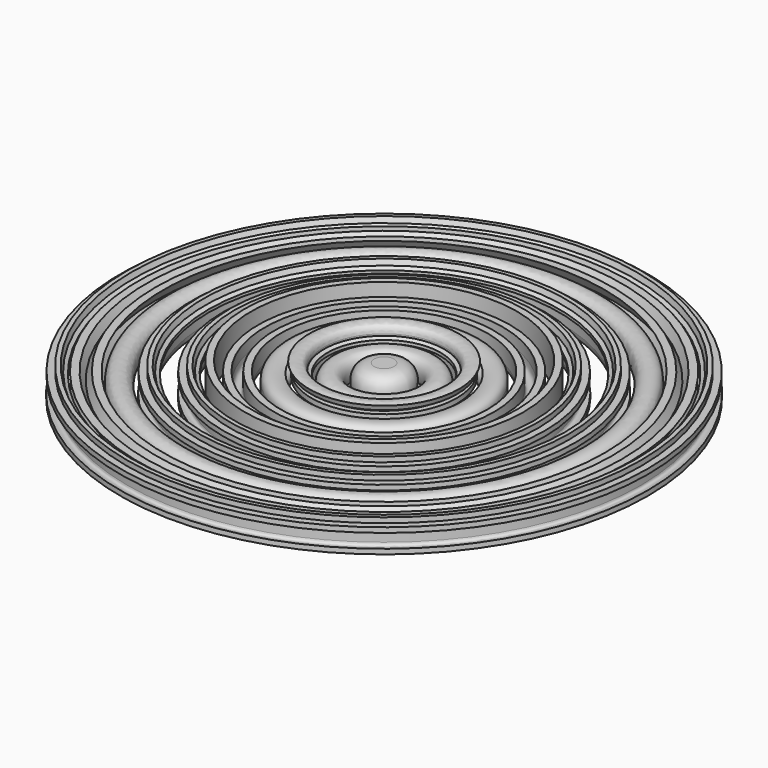
from build123d import *

# Parameters (mm, degrees)
F0_TEXT_SIZE = 64.0149060119
F1_DEPTH     = 25.4
F1_FACE_W    = 9.5322195983
F1_FACE_H    = 48.64132624


# Not quite as in the source:
# - Text() gives the source's letters only with a copy of the font that has no kerning and outlines rounded to 1/6400 em; it was checked with that copy


with BuildPart() as f1:
    # F0 (on Front) → F1 (new body)
    with BuildSketch(Plane.XZ):
        with Locations((-95.4079255462, 3.5789469257)):
            Text('Default text', F0_TEXT_SIZE, font='Open Sans', font_style=FontStyle.BOLD, text_align=(TextAlign.LEFT, TextAlign.BOTTOM))
    extrude(amount=F1_DEPTH)


with BuildPart() as f2:
    # F1_face (on face) → F2 (revolve)
    with BuildSketch(Plane(origin=(-72.8163367303, 0, 26.4794588541), x_dir=(1, 0, 0), z_dir=(0, 1, 0))):
        with BuildLine():
            add(Edge.make_bspline(
                [(-3.8972357946, 22.9005119284), (8.2255870314, 22.9005119284), (21.0785798791, 10.8977170511), (21.0785798791, -10.9873789417), (8.6956964974, -22.8001295667), (-2.4969097256, -22.8001295667)],
                knots=[0, 0, 0, 1, 2, 2.9397163121, 3.8794326241, 3.8794326241, 3.8794326241], degree=2))
            Line((-3.8972357946, 22.9005119284), (-16.8402496039, 22.9005119284))
            Line((-16.8402496039, 22.9005119284), (-16.8402496039, -22.8001295667))
            Line((-16.8402496039, -22.8001295667), (-2.4969097256, -22.8001295667))
        make_face()
        with BuildLine():
            Line((-7.1479927405, 14.8986486769), (-2.9970261788, 14.8986486769))
            add(Edge.make_bspline(
                [(-1.9967932724, -14.8582802896), (11.0062345113, -14.8582802896), (11.0062345113, 14.8986486769), (-2.9970261788, 14.8986486769)],
                knots=[0, 0, 0, 1, 2.0210597826, 2.0210597826, 2.0210597826], degree=2))
            Line((-1.9967932724, -14.8582802896), (-7.1479927405, -14.8582802896))
            Line((-7.1479927405, -14.8582802896), (-7.1479927405, 14.8986486769))
        make_face(mode=Mode.SUBTRACT)
    revolve(axis=Axis((-89.6565863342, 0, 26.4292676732), (0, 0, 1)))


with BuildPart() as f2b:
    # F1_face (on face) → F2, piece 2 (revolve)
    with BuildSketch(Plane(origin=(-72.8163367303, 0, 26.4794588541), x_dir=(1, 0, 0), z_dir=(0, 1, 0))):
        with BuildLine():
            add(Edge.make_bspline(
                [(59.8676119907, 3.1759190134), (59.8676119907, -4.2658138104), (51.6156905126, -12.6977772117), (36.4621619801, -12.6977772117), (27.6801170616, -3.105543639), (27.6801170616, 14.2084879714), (37.1823296727, 23.5306586594), (49.7152479904, 23.5306586594), (55.396570899, 22.3103745136), (57.897153165, 21.0600833805)],
                knots=[0, 0, 0, 1, 2, 3.0472972973, 4.0945945946, 5.1120713538, 6.129548113, 6.6244063233, 7.1192645336, 7.1192645336, 7.1192645336], degree=2))
            Line((59.8676119907, 3.1759190134), (59.8676119907, 7.8069973702))
            Line((59.8676119907, 7.8069973702), (37.3323646087, 7.8069973702))
            add(Edge.make_bspline(
                [(57.897153165, 13.678364531), (54.8364404713, 15.1186999163), (49.2151315372, 16.4290050237), (41.9934499527, 16.4290050237), (37.4924018737, 11.8679429704), (37.3323646087, 7.8069973702)],
                knots=[0, 0, 0, 1, 2, 3.2848101266, 4.5696202532, 4.5696202532, 4.5696202532], degree=2))
            Line((57.897153165, 13.678364531), (57.897153165, 21.0600833805))
        make_face()
        with BuildLine():
            add(Edge.make_bspline(
                [(37.5524158481, 1.4555184144), (37.8024740747, -2.0753037453), (41.2432752729, -5.9161981061), (47.3046866859, -5.9161981061), (50.8655158328, -2.0753037453), (50.9355321362, 1.4555184144)],
                knots=[0, 0, 0, 1, 2, 3, 4, 4, 4], degree=2))
            Line((37.5524158481, 1.4555184144), (50.9355321362, 1.4555184144))
        make_face(mode=Mode.SUBTRACT)
    revolve(axis=Axis((-89.6565863342, 0, 26.4292676732), (0, 0, 1)))


with BuildPart() as f2c:
    # F1_face (on face) → F2, piece 3 (revolve)
    with BuildSketch(Plane(origin=(-72.8163367303, 0, 26.4794588541), x_dir=(1, 0, 0), z_dir=(0, 1, 0))):
        with BuildLine():
            Line((86.9339144389, -4.8859582124), (78.6819929608, -4.8859582124))
            Line((78.6819929608, -4.8859582124), (78.6819929608, 22.9005119284))
            Line((78.6819929608, 22.9005119284), (69.1497733625, 22.9005119284))
            Line((69.1497733625, 22.9005119284), (69.1497733625, -4.8859582124))
            Line((69.1497733625, -4.8859582124), (63.8985506037, -4.8859582124))
            Line((63.8985506037, -4.8859582124), (63.8985506037, -9.487029582))
            Line((63.8985506037, -9.487029582), (69.1497733625, -12.0476258225))
            Line((69.1497733625, -12.0476258225), (69.1497733625, -14.608222063))
            add(Edge.make_bspline(
                [(90.2846946755, -24.6105511274), (86.4337979857, -26.0808934998), (75.0311428523, -26.0808934998), (69.1497733625, -20.5796125144), (69.1497733625, -14.608222063)],
                knots=[0, 0, 0, 1, 2.3123732252, 3.6247464503, 3.6247464503, 3.6247464503], degree=2))
            Line((90.2846946755, -24.6105511274), (87.8441263838, -17.6089207823))
            add(Edge.make_bspline(
                [(78.6819929608, -14.2381358876), (78.6819929608, -16.1085714226), (80.5024168505, -18.5191327272), (84.9634556132, -18.5191327272), (87.8441263838, -17.6089207823)],
                knots=[0, 0, 0, 1, 2, 3.197044335, 3.197044335, 3.197044335], degree=2))
            Line((78.6819929608, -14.2381358876), (78.6819929608, -12.0476258225))
            Line((78.6819929608, -12.0476258225), (86.9339144389, -12.0476258225))
            Line((86.9339144389, -12.0476258225), (86.9339144389, -4.8859582124))
        make_face()
    revolve(axis=Axis((-89.6565863342, 0, 26.4292676732), (0, 0, 1)))


with BuildPart() as f2d:
    # F1_face (on face) → F2, piece 4 (revolve)
    with BuildSketch(Plane(origin=(-72.8163367303, 0, 26.4794588541), x_dir=(1, 0, 0), z_dir=(0, 1, 0))):
        with BuildLine():
            Line((114.6003566309, 22.9005119284), (112.749925754, 18.1494056228))
            Line((112.749925754, 18.1494056228), (112.4998675274, 18.1494056228))
            add(Edge.make_bspline(
                [(105.7182884218, 1.3354904656), (97.8764624353, 1.6155556794), (90.0946504232, 6.8967854254), (90.0946504232, 17.7693171184), (95.8759966224, 23.5306586594), (104.9981207291, 23.5306586594), (110.099308552, 21.1801113293), (112.4998675274, 18.1494056228)],
                knots=[0, 0, 0, 1, 2, 2.9550359712, 3.9100719424, 4.6866320065, 5.4631920706, 5.4631920706, 5.4631920706], degree=2))
            Line((105.7182884218, 1.3354904656), (111.7897021638, 1.1454462134))
            Line((111.7897021638, 1.1454462134), (111.7897021638, -0.3849101335))
            add(Edge.make_bspline(
                [(96.4961410244, -3.1655576134), (102.1574592749, -5.6961468666), (111.7897021638, -5.6961468666), (111.7897021638, -0.3849101335)],
                knots=[0, 0, 0, 1, 2.2983293556, 2.2983293556, 2.2983293556], degree=2))
            Line((96.4961410244, -3.1655576134), (93.3454073692, -9.6070575308))
            add(Edge.make_bspline(
                [(121.2519054587, -0.3849101335), (121.2519054587, -6.6363657987), (113.7501586605, -12.7677935151), (99.376811795, -12.7677935151), (93.3454073692, -9.6070575308)],
                knots=[0, 0, 0, 1, 2, 3.0440967283, 3.0440967283, 3.0440967283], degree=2))
            Line((121.2519054587, -0.3849101335), (121.2519054587, 22.9005119284))
            Line((121.2519054587, 22.9005119284), (114.6003566309, 22.9005119284))
        make_face()
        with BuildLine():
            Line((111.7897021638, 6.7067411732), (108.0988427391, 6.836771451))
            add(Edge.make_bspline(
                [(111.7897021638, 9.5874119437), (111.7897021638, 12.738145599), (107.8187775253, 16.5590353016), (99.8769282482, 16.5590353016), (99.8769282482, 9.7074398925), (103.9378738483, 6.9567993998), (108.0988427391, 6.836771451)],
                knots=[0, 0, 0, 1, 2, 3.3915662651, 4.3594626029, 5.3273589407, 5.3273589407, 5.3273589407], degree=2))
            Line((111.7897021638, 9.5874119437), (111.7897021638, 6.7067411732))
        make_face(mode=Mode.SUBTRACT)
    revolve(axis=Axis((-89.6565863342, 0, 26.4292676732), (0, 0, 1)))


with BuildPart() as f2e:
    # F1_face (on face) → F2, piece 5 (revolve)
    with BuildSketch(Plane(origin=(-72.8163367303, 0, 26.4794588541), x_dir=(1, 0, 0), z_dir=(0, 1, 0))):
        with BuildLine():
            Line((155.8299570342, 22.9005119284), (154.549658914, 18.4294708366))
            Line((154.549658914, 18.4294708366), (154.0495424608, 18.4294708366))
            add(Edge.make_bspline(
                [(130.8841483477, 10.7376797861), (130.8841483477, 16.929121477), (137.1356040129, 23.5306586594), (146.8878748507, 23.5306586594), (152.5191861139, 20.8700391283), (154.0495424608, 18.4294708366)],
                knots=[0, 0, 0, 1, 2, 2.5827922078, 3.1655844156, 3.1655844156, 3.1655844156], degree=2))
            Line((130.8841483477, 10.7376797861), (130.8841483477, -12.0476258225))
            Line((130.8841483477, -12.0476258225), (140.4163679461, -12.0476258225))
            Line((140.4163679461, -12.0476258225), (140.4163679461, 8.3671277979))
            add(Edge.make_bspline(
                [(153.609439982, 4.3962031593), (153.609439982, 10.5876448501), (150.048610835, 15.9288885705), (143.1069944644, 15.9288885705), (140.4163679461, 12.1480081842), (140.4163679461, 8.3671277979)],
                knots=[0, 0, 0, 1, 2, 2.735, 3.47, 3.47, 3.47], degree=2))
            Line((153.609439982, 4.3962031593), (153.609439982, -12.0476258225))
            Line((153.609439982, -12.0476258225), (163.1416595803, -12.0476258225))
            Line((163.1416595803, -12.0476258225), (163.1416595803, 22.9005119284))
            Line((163.1416595803, 22.9005119284), (155.8299570342, 22.9005119284))
        make_face()
    revolve(axis=Axis((-89.6565863342, 0, 26.4292676732), (0, 0, 1)))


with BuildPart() as f2f:
    # F1_face (on face) → F2, piece 6 (revolve)
    with BuildSketch(Plane(origin=(-72.8163367303, 0, 26.4794588541), x_dir=(1, 0, 0), z_dir=(0, 1, 0))):
        with Locations((177.9100984438, -1.4201511916)):
            Rectangle(F1_FACE_W, F1_FACE_H)
    revolve(axis=Axis((-89.6565863342, 0, 26.4292676732), (0, 0, 1)))


with BuildPart() as f2g:
    # F1_face (on face) → F2, piece 7 (revolve)
    with BuildSketch(Plane(origin=(-72.8163367303, 0, 26.4794588541), x_dir=(1, 0, 0), z_dir=(0, 1, 0))):
        with BuildLine():
            add(Edge.make_bspline(
                [(213.4033631287, 14.8386347025), (209.9025479562, 15.9288885705), (205.521527826, 15.9288885705), (203.2409967993, 13.988436732), (203.2409967993, 11.957963932)],
                knots=[0, 0, 0, 1, 1.752, 2.504, 2.504, 2.504], degree=2))
            Line((213.4033631287, 14.8386347025), (213.4033631287, 21.9302860091))
            add(Edge.make_bspline(
                [(193.708777201, 11.957963932), (193.708777201, 17.7393101312), (198.9299929726, 23.5306586594), (209.8425339818, 23.5306586594), (213.4033631287, 21.9302860091)],
                knots=[0, 0, 0, 1, 2, 2.9073426573, 2.9073426573, 2.9073426573], degree=2))
            Line((193.708777201, 11.957963932), (193.708777201, -4.8859582124))
            Line((193.708777201, -4.8859582124), (189.1477151476, -4.8859582124))
            Line((189.1477151476, -4.8859582124), (189.1477151476, -8.9168968254))
            Line((189.1477151476, -8.9168968254), (194.3989379064, -12.1076397969))
            Line((194.3989379064, -12.1076397969), (197.1495783991, -19.4893586464))
            Line((197.1495783991, -19.4893586464), (203.2409967993, -19.4893586464))
            Line((203.2409967993, -19.4893586464), (203.2409967993, -12.0476258225))
            Line((203.2409967993, -12.0476258225), (213.0232746243, -12.0476258225))
            Line((213.0232746243, -12.0476258225), (213.0232746243, -4.8859582124))
            Line((213.0232746243, -4.8859582124), (203.2409967993, -4.8859582124))
            Line((203.2409967993, -4.8859582124), (203.2409967993, 11.957963932))
        make_face()
    revolve(axis=Axis((-89.6565863342, 0, 26.4292676732), (0, 0, 1)))


with BuildPart() as f2h:
    # F1_face (on face) → F2, piece 8 (revolve)
    with BuildSketch(Plane(origin=(-72.8163367303, 0, 26.4794588541), x_dir=(1, 0, 0), z_dir=(0, 1, 0))):
        with BuildLine():
            add(Edge.make_bspline(
                [(257.8237065036, 14.8386347025), (254.322891331, 15.9288885705), (249.9418712009, 15.9288885705), (247.6613401742, 13.988436732), (247.6613401742, 11.957963932)],
                knots=[0, 0, 0, 1, 1.752, 2.504, 2.504, 2.504], degree=2))
            Line((257.8237065036, 14.8386347025), (257.8237065036, 21.9302860091))
            add(Edge.make_bspline(
                [(238.1291205758, 11.957963932), (238.1291205758, 17.7393101312), (243.3503363474, 23.5306586594), (254.2628773567, 23.5306586594), (257.8237065036, 21.9302860091)],
                knots=[0, 0, 0, 1, 2, 2.9073426573, 2.9073426573, 2.9073426573], degree=2))
            Line((238.1291205758, 11.957963932), (238.1291205758, -4.8859582124))
            Line((238.1291205758, -4.8859582124), (233.5680585225, -4.8859582124))
            Line((233.5680585225, -4.8859582124), (233.5680585225, -8.9168968254))
            Line((233.5680585225, -8.9168968254), (238.8192812813, -12.1076397969))
            Line((238.8192812813, -12.1076397969), (241.569921774, -19.4893586464))
            Line((241.569921774, -19.4893586464), (247.6613401742, -19.4893586464))
            Line((247.6613401742, -19.4893586464), (247.6613401742, -12.0476258225))
            Line((247.6613401742, -12.0476258225), (257.4436179991, -12.0476258225))
            Line((257.4436179991, -12.0476258225), (257.4436179991, -4.8859582124))
            Line((257.4436179991, -4.8859582124), (247.6613401742, -4.8859582124))
            Line((247.6613401742, -4.8859582124), (247.6613401742, 11.957963932))
        make_face()
    revolve(axis=Axis((-89.6565863342, 0, 26.4292676732), (0, 0, 1)))


with BuildPart() as f2i:
    # F1_face (on face) → F2, piece 9 (revolve)
    with BuildSketch(Plane(origin=(-72.8163367303, 0, 26.4794588541), x_dir=(1, 0, 0), z_dir=(0, 1, 0))):
        with BuildLine():
            add(Edge.make_bspline(
                [(294.9523519905, 3.1759190134), (294.9523519905, -4.2658138104), (286.7004305124, -12.6977772117), (271.5469019799, -12.6977772117), (262.7648570614, -3.105543639), (262.7648570614, 14.2084879714), (272.2670696725, 23.5306586594), (284.7999879902, 23.5306586594), (290.4813108987, 22.3103745136), (292.9818931648, 21.0600833805)],
                knots=[0, 0, 0, 1, 2, 3.0472972973, 4.0945945946, 5.1120713538, 6.129548113, 6.6244063233, 7.1192645336, 7.1192645336, 7.1192645336], degree=2))
            Line((294.9523519905, 3.1759190134), (294.9523519905, 7.8069973702))
            Line((294.9523519905, 7.8069973702), (272.4171046085, 7.8069973702))
            add(Edge.make_bspline(
                [(292.9818931648, 13.678364531), (289.9211804711, 15.1186999163), (284.2998715369, 16.4290050237), (277.0781899525, 16.4290050237), (272.5771418735, 11.8679429704), (272.4171046085, 7.8069973702)],
                knots=[0, 0, 0, 1, 2, 3.2848101266, 4.5696202532, 4.5696202532, 4.5696202532], degree=2))
            Line((292.9818931648, 13.678364531), (292.9818931648, 21.0600833805))
        make_face()
        with BuildLine():
            add(Edge.make_bspline(
                [(272.6371558479, 1.4555184144), (272.8872140745, -2.0753037453), (276.3280152726, -5.9161981061), (282.3894266857, -5.9161981061), (285.9502558326, -2.0753037453), (286.020272136, 1.4555184144)],
                knots=[0, 0, 0, 1, 2, 3, 4, 4, 4], degree=2))
            Line((272.6371558479, 1.4555184144), (286.020272136, 1.4555184144))
        make_face(mode=Mode.SUBTRACT)
    revolve(axis=Axis((-89.6565863342, 0, 26.4292676732), (0, 0, 1)))


with BuildPart() as f2j:
    # F1_face (on face) → F2, piece 10 (revolve)
    with BuildSketch(Plane(origin=(-72.8163367303, 0, 26.4794588541), x_dir=(1, 0, 0), z_dir=(0, 1, 0))):
        Polygon((309.8658246255, 5.0563568775), (298.6132044281, -12.0476258225), (309.4257221466, -12.0476258225), (316.2073012523, -0.9150335739), (323.0488943323, -12.0476258225), (333.8714143799, -12.0476258225), (322.4887639047, 5.0563568775), (334.4015378204, 22.9005119284), (323.5490107855, 22.9005119284), (316.2073012523, 10.9277240383), (308.8355847318, 22.9005119284), (298.0130646842, 22.9005119284), align=None)
    revolve(axis=Axis((-89.6565863342, 0, 26.4292676732), (0, 0, 1)))


with BuildPart() as f2k:
    # F1_face (on face) → F2, piece 11 (revolve)
    with BuildSketch(Plane(origin=(-72.8163367303, 0, 26.4794588541), x_dir=(1, 0, 0), z_dir=(0, 1, 0))):
        with BuildLine():
            add(Edge.make_bspline(
                [(360.4376003749, 14.8386347025), (356.9367852024, 15.9288885705), (352.5557650722, 15.9288885705), (350.2752340455, 13.988436732), (350.2752340455, 11.957963932)],
                knots=[0, 0, 0, 1, 1.752, 2.504, 2.504, 2.504], degree=2))
            Line((360.4376003749, 14.8386347025), (360.4376003749, 21.9302860091))
            add(Edge.make_bspline(
                [(340.7430144472, 11.957963932), (340.7430144472, 17.7393101312), (345.9642302188, 23.5306586594), (356.876771228, 23.5306586594), (360.4376003749, 21.9302860091)],
                knots=[0, 0, 0, 1, 2, 2.9073426573, 2.9073426573, 2.9073426573], degree=2))
            Line((340.7430144472, 11.957963932), (340.7430144472, -4.8859582124))
            Line((340.7430144472, -4.8859582124), (336.1819523938, -4.8859582124))
            Line((336.1819523938, -4.8859582124), (336.1819523938, -8.9168968254))
            Line((336.1819523938, -8.9168968254), (341.4331751526, -12.1076397969))
            Line((341.4331751526, -12.1076397969), (344.1838156453, -19.4893586464))
            Line((344.1838156453, -19.4893586464), (350.2752340455, -19.4893586464))
            Line((350.2752340455, -19.4893586464), (350.2752340455, -12.0476258225))
            Line((350.2752340455, -12.0476258225), (360.0575118704, -12.0476258225))
            Line((360.0575118704, -12.0476258225), (360.0575118704, -4.8859582124))
            Line((360.0575118704, -4.8859582124), (350.2752340455, -4.8859582124))
            Line((350.2752340455, -4.8859582124), (350.2752340455, 11.957963932))
        make_face()
    revolve(axis=Axis((-89.6565863342, 0, 26.4292676732), (0, 0, 1)))


solid = Compound([f2.part, f2b.part, f2c.part, f2d.part, f2e.part, f2f.part, f2g.part, f2h.part, f2i.part, f2j.part, f2k.part])
